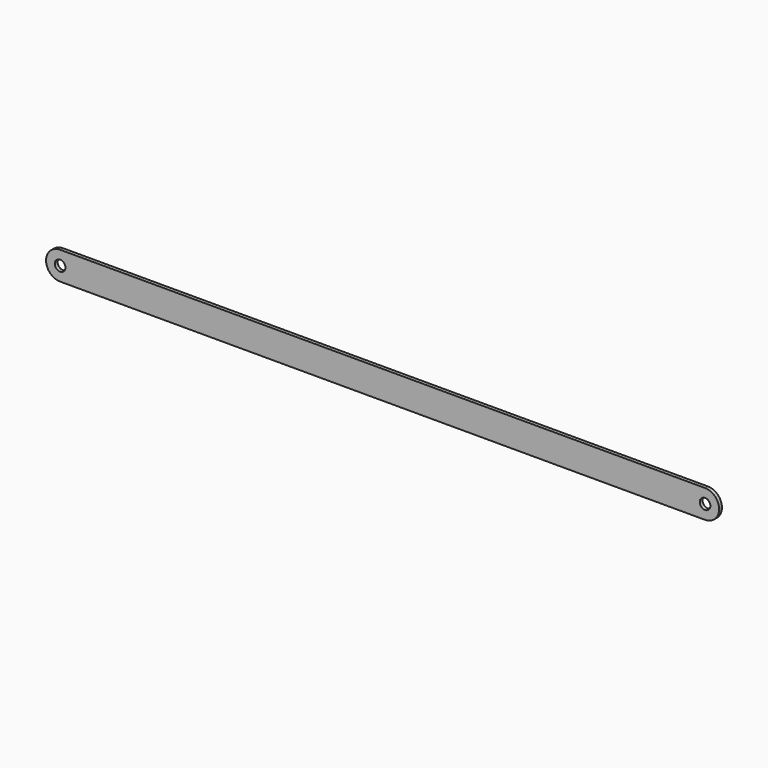
from build123d import *

# Parameters (mm, degrees)
F0_W     = 609.6
F0_H     = 25.4
F1_DEPTH = 3.175
F2_R     = 12.69999
F3_R     = 4.8006
F4_DEPTH = 3.175


# Not quite as in the source:
# - a fillet or chamfer is up to 0.001 mm smaller than in the source, because OpenCascade refuses the exact size


with BuildPart() as f1:
    # F0 (on Front) → F1 (new body)
    with BuildSketch(Plane.XZ):
        with Locations((-378.0265757293, 35.5002675663)):
            Rectangle(F0_W, F0_H)
    extrude(amount=F1_DEPTH)

    # F2 (radius 12.7 in the source; OpenCascade refuses exactly that, so slightly less here)
    f2_edges = [f1.edges().sort_by_distance(p)[0] for p in [
        (-73.226576, -1.5875, 48.200268),
        (-73.226576, -1.5875, 22.800268),
        (-682.826576, -1.5875, 48.200268),
        (-682.826576, -1.5875, 22.800268),
    ]]
    fillet(f2_edges, radius=F2_R)

    # F3 (on face) → F4 (cut)
    with BuildSketch(Plane.XZ.offset(3.175)):
        with Locations((-670.1265757293, 35.5002675663)):
            Circle(F3_R)
        with Locations((-85.9265757293, 35.5002675663)):
            Circle(F3_R)
    extrude(amount=-F4_DEPTH, mode=Mode.SUBTRACT)


solid = f1.part
